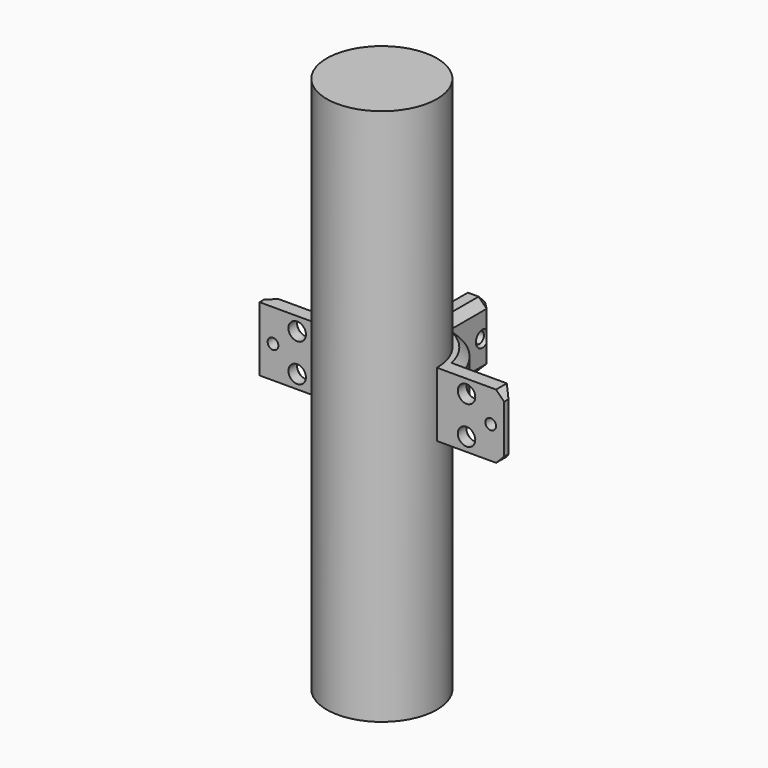
from build123d import *

# Parameters (mm, degrees)
F0_R     = 10.25
F1_DEPTH = 50
F3_DEPTH = 6
F4_R     = 1.625
F5_DEPTH = 12.5
F4_R_2   = 1
F6_DEPTH = 12.5
F7_COUNT = 4
F10_SIZE = 1.49999


# Not quite as in the source:
# - a fillet or chamfer that OpenCascade refuses, or shapes differently, is made with other operations: its cross-section is extruded or revolved along the edge and cut away or added
# - a fillet or chamfer is up to 0.001 mm smaller than in the source, because OpenCascade refuses the exact size


with BuildPart() as f1:
    # F0 (on Top) → F1 (new body, symmetric)
    with BuildSketch(Plane.XY):
        Circle(F0_R)
    extrude(amount=F1_DEPTH, both=True)


with BuildPart() as f3:
    # F2 (on Top) → F3 (new body, symmetric)
    with BuildSketch(Plane.XY):
        with BuildLine():
            Line((-2.5, 22.75), (-2.5, 12.50249975))
            ThreePointArc((-2.5, 12.50249975), (-1.2561107011, 12.6879740663), (0, 12.75))
            Line((0, 12.75), (0, 22.75))
            Line((0, 22.75), (-2.5, 22.75))
        make_face()
        with BuildLine():
            ThreePointArc((0, 12.75), (1.2561107011, 12.6879740663), (2.5, 12.50249975))
            Line((2.5, 12.50249975), (2.5, 22.75))
            Line((2.5, 22.75), (0, 22.75))
            Line((0, 22.75), (0, 12.75))
        make_face()
        with BuildLine():
            Line((-12.75, 0), (-10.25, 0))
            ThreePointArc((-10.25, 0), (0, 10.25), (10.25, 0))
            Line((10.25, 0), (12.75, 0))
            ThreePointArc((12.75, 0), (12.6879740663, 1.2561107011), (12.50249975, 2.5))
            ThreePointArc((12.50249975, 2.5), (11.7416340406, 4.9695603484), (10.4984525255, 7.2349840753))
            ThreePointArc((10.4984525255, 7.2349840753), (9.7975676461, 8.1590543705), (9.0156114601, 9.0156114601))
            ThreePointArc((9.0156114601, 9.0156114601), (8.0063926665, 9.9227101373), (6.9064852098, 10.7174139627))
            ThreePointArc((6.9064852098, 10.7174139627), (4.7871832864, 11.817164473), (2.5, 12.50249975))
            ThreePointArc((2.5, 12.50249975), (1.2561107011, 12.6879740663), (0, 12.75))
            ThreePointArc((0, 12.75), (-1.2561107011, 12.6879740663), (-2.5, 12.50249975))
            ThreePointArc((-2.5, 12.50249975), (-4.7871832864, 11.817164473), (-6.9064852098, 10.7174139627))
            ThreePointArc((-6.9064852098, 10.7174139627), (-8.0063926665, 9.9227101373), (-9.0156114601, 9.0156114601))
            ThreePointArc((-9.0156114601, 9.0156114601), (-9.7975676461, 8.1590543705), (-10.4984525255, 7.2349840753))
            ThreePointArc((-10.4984525255, 7.2349840753), (-11.7416340406, 4.9695603484), (-12.50249975, 2.5))
            ThreePointArc((-12.50249975, 2.5), (-12.6879740663, 1.2561107011), (-12.75, 0))
        make_face()
        with BuildLine():
            ThreePointArc((12.50249975, 2.5), (12.6879740663, 1.2561107011), (12.75, 0))
            Line((12.75, 0), (22.75, 0))
            Line((22.75, 0), (22.75, 2.5))
            Line((22.75, 2.5), (12.50249975, 2.5))
        make_face()
        with BuildLine():
            Line((-22.75, 0), (-12.75, 0))
            ThreePointArc((-12.75, 0), (-12.6879740663, 1.2561107011), (-12.50249975, 2.5))
            Line((-12.50249975, 2.5), (-22.75, 2.5))
            Line((-22.75, 2.5), (-22.75, 0))
        make_face()
    extrude(amount=F3_DEPTH, both=True)

    # F4 (on face) → F5 (cut, symmetric)
    with BuildSketch(Plane.XZ):
        with Locations((-15.75, 3.5)):
            Circle(F4_R)
        with Locations((-15.75, -3.5)):
            Circle(F4_R)
        with Locations((15.75, 3.5)):
            Circle(F4_R)
        with Locations((15.75, -3.5)):
            Circle(F4_R)
    extrude(amount=F5_DEPTH, both=True, mode=Mode.SUBTRACT)


with BuildPart() as f6:
    # F4 (on face) → F6 (new body, symmetric)
    with BuildSketch(Plane.XZ):
        with Locations((-20.25, 0)):
            Circle(F4_R_2)
    extrude(amount=F6_DEPTH, both=True)


with BuildPart() as f7_1:
    # F7: instance of F6
    add(f6.part.rotate(Axis((0, 0, 50), (0, 0, 1)), 1 * 360 / F7_COUNT))


with BuildPart() as f7_2:
    # F7: instance of F6
    add(f6.part.rotate(Axis((0, 0, 50), (0, 0, 1)), 2 * 360 / F7_COUNT))


with BuildPart() as f7_3:
    # F7: instance of F6
    add(f6.part.rotate(Axis((0, 0, 50), (0, 0, 1)), 3 * 360 / F7_COUNT))


with BuildPart() as f3_1:
    add(f3.part)

    # F9: cut F7_3, F6, F7_2
    add(f7_3.part, mode=Mode.SUBTRACT)
    add(f6.part, mode=Mode.SUBTRACT)
    add(f7_2.part, mode=Mode.SUBTRACT)

    # F10 (size 1.5 in the source; OpenCascade refuses exactly that, so slightly less here)
    f10_edges = [f3_1.edges().sort_by_distance(p)[0] for p in [
        (22.75, 1.25, 6),
        (22.75, 1.25, -6),
        (0, 22.75, -6),
        (0, 22.75, 6),
        (2.5, 17.62625, 6),
        (-2.5, 17.62625, 6),
        (9.015611, 9.015611, 6),
        (-9.015611, 9.015611, 6),
        (-9.015611, 9.015611, -6),
        (-2.5, 17.62625, -6),
        (2.5, 17.62625, -6),
        (9.015611, 9.015611, -6),
        (-2.5, 22.75, 0),
        (2.5, 22.75, 0),
        (-22.75, 2.5, 0),
        (22.75, 2.5, 0),
    ]]
    chamfer(f10_edges, length=F10_SIZE)

    # F11: chamfer of 0.5 on 8 edges, made by hand

    # F11_s1 → F11_t2 (revolve, cut)
    with BuildSketch(Plane.XY):
        Polygon((18.75, 2.5), (19.25, 2), (19.25, 2.5), align=None)
    revolve(axis=Axis((20.25, 2.5, 0), (0, 1, 0)), mode=Mode.SUBTRACT)

    # F11_s3 → F11_t4 (revolve, cut)
    with BuildSketch(Plane.XY):
        Polygon((2.5, 18.75), (2, 19.25), (2.5, 19.25), align=None)
    revolve(axis=Axis((2.5, 20.25, 0), (-1, 0, 0)), mode=Mode.SUBTRACT)

    # F11_s5 → F11_t6 (revolve, cut)
    with BuildSketch(Plane.XY):
        Polygon((-2, 19.25), (-2.5, 18.75), (-2.5, 19.25), align=None)
    revolve(axis=Axis((-2.5, 20.25, 0), (-1, 0, 0)), mode=Mode.SUBTRACT)

    # F11_s7 → F11_t8 (revolve, cut)
    with BuildSketch(Plane.XY.offset(3.5)):
        Polygon((17.875, 2.5), (17.375, 2), (17.375, 2.5), align=None)
    revolve(axis=Axis((15.75, 2.5, 3.5), (0, -1, 0)), mode=Mode.SUBTRACT)

    # F11_s9 → F11_t10 (revolve, cut)
    with BuildSketch(Plane.XY.offset(-3.5)):
        Polygon((17.875, 2.5), (17.375, 2), (17.375, 2.5), align=None)
    revolve(axis=Axis((15.75, 2.5, -3.5), (0, -1, 0)), mode=Mode.SUBTRACT)

    # F11_s11 → F11_t12 (revolve, cut)
    with BuildSketch(Plane.XY.offset(-3.5)):
        Polygon((-13.625, 2.5), (-14.125, 2), (-14.125, 2.5), align=None)
    revolve(axis=Axis((-15.75, 2.5, -3.5), (0, -1, 0)), mode=Mode.SUBTRACT)

    # F11_s13 → F11_t14 (revolve, cut)
    with BuildSketch(Plane.XY.offset(3.5)):
        Polygon((-13.625, 2.5), (-14.125, 2), (-14.125, 2.5), align=None)
    revolve(axis=Axis((-15.75, 2.5, 3.5), (0, -1, 0)), mode=Mode.SUBTRACT)

    # F11_s15 → F11_t16 (revolve, cut)
    with BuildSketch(Plane.XY):
        Polygon((-18.75, 2.5), (-19.25, 2), (-19.25, 2.5), align=None)
    revolve(axis=Axis((-20.25, 2.5, 0), (0, -1, 0)), mode=Mode.SUBTRACT)


solid = Compound([f1.part, f3_1.part])
